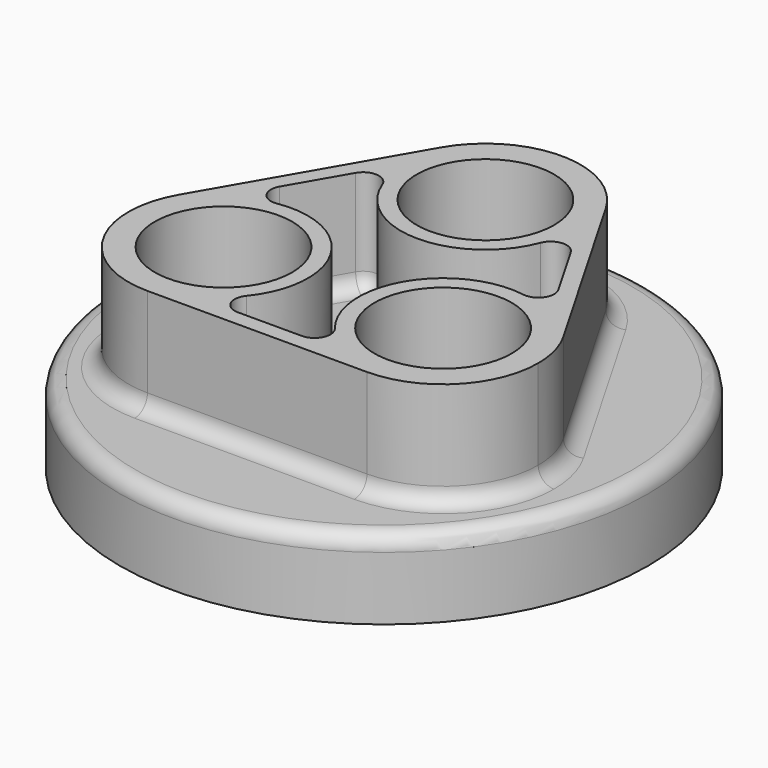
from build123d import *

# Parameters (mm, degrees)
F0_R         = 50
F0_R_2       = 13
F1_DEPTH     = 15
F2_T         = -2.5
F3_DEPTH     = 20
F4_T         = 3
F4_T3_DEPTH  = 47.5692193817
F4_T5_DEPTH  = 47.5692193817
F4_T7_DEPTH  = 47.5692193817
F4_T18_ANGLE = 120.000000001
F4_T20_ANGLE = 120.000000001
F4_T22_ANGLE = 120.000000001
F5_R         = 3


# Not quite as in the source:
# - two fillets or chamfers of one size are made in one step
# - a shell that OpenCascade refuses in one call is made with other operations: the cavity is built on its own and cut out


with BuildPart() as f1:
    # F0 (on Top) → F1 (new body)
    with BuildSketch(Plane.XY):
        Circle(F0_R)
        with BuildLine():
            ThreePointArc((-20.7846096908, -30), (-36.3730669589, -21), (-36.3730669589, -3))
            Line((-36.3730669589, -3), (-15.5884572681, 33))
            ThreePointArc((-15.5884572681, 33), (0, 42), (15.5884572681, 33))
            Line((15.5884572681, 33), (36.3730669589, -3))
            ThreePointArc((36.3730669589, -3), (38.171274564, -7.3412571882), (38.7846096908, -12))
            ThreePointArc((38.7846096908, -12), (33.5125317522, -24.7279220614), (20.7846096908, -30))
            Line((20.7846096908, -30), (-20.7846096908, -30))
        make_face(mode=Mode.SUBTRACT)
        with BuildLine():
            ThreePointArc((-20.7846096908, -30), (-8.0566876295, -24.7279220614), (-2.7846096908, -12))
            ThreePointArc((-2.7846096908, -12), (-16.125866879, 5.3866648732), (-36.3730669589, -3))
            ThreePointArc((-36.3730669589, -3), (-36.3730669589, -21), (-20.7846096908, -30))
        make_face()
        with Locations((-20.7846096908, -12)):
            Circle(F0_R_2, mode=Mode.SUBTRACT)
        with BuildLine():
            ThreePointArc((15.5884572681, 33), (0, 42), (-15.5884572681, 33))
            ThreePointArc((-15.5884572681, 33), (-4.6587428118, 6.6133351268), (18, 24))
            ThreePointArc((18, 24), (17.3866648732, 28.6587428118), (15.5884572681, 33))
        make_face()
        with Locations((0, 24)):
            Circle(F0_R_2, mode=Mode.SUBTRACT)
        with BuildLine():
            ThreePointArc((36.3730669589, -3), (5.1961524227, -3), (20.7846096908, -30))
            ThreePointArc((20.7846096908, -30), (33.5125317522, -24.7279220614), (38.7846096908, -12))
            ThreePointArc((38.7846096908, -12), (38.171274564, -7.3412571882), (36.3730669589, -3))
        make_face()
        with Locations((20.7846096908, -12)):
            Circle(F0_R_2, mode=Mode.SUBTRACT)
        with BuildLine():
            ThreePointArc((-36.3730669589, -3), (-16.125866879, 5.3866648732), (-2.7846096908, -12))
            ThreePointArc((-2.7846096908, -12), (-8.0566876295, -24.7279220614), (-20.7846096908, -30))
            Line((-20.7846096908, -30), (20.7846096908, -30))
            ThreePointArc((20.7846096908, -30), (5.1961524227, -3), (36.3730669589, -3))
            Line((36.3730669589, -3), (15.5884572681, 33))
            ThreePointArc((15.5884572681, 33), (17.3866648732, 28.6587428118), (18, 24))
            ThreePointArc((18, 24), (-4.6587428118, 6.6133351268), (-15.5884572681, 33))
            Line((-15.5884572681, 33), (-36.3730669589, -3))
        make_face()
    extrude(amount=-F1_DEPTH)

    # F2
    f2_openings = [f1.faces().sort_by_distance(p)[0] for p in [
        (0, 0, -15),
    ]]
    offset(amount=F2_T, openings=f2_openings)

    # F0 (on Top) → F3 (join)
    with BuildSketch(Plane.XY):
        with BuildLine():
            ThreePointArc((15.5884572681, 33), (0, 42), (-15.5884572681, 33))
            ThreePointArc((-15.5884572681, 33), (-4.6587428118, 6.6133351268), (18, 24))
            ThreePointArc((18, 24), (17.3866648732, 28.6587428118), (15.5884572681, 33))
        make_face()
        with Locations((0, 24)):
            Circle(F0_R_2, mode=Mode.SUBTRACT)
        with BuildLine():
            ThreePointArc((-20.7846096908, -30), (-8.0566876295, -24.7279220614), (-2.7846096908, -12))
            ThreePointArc((-2.7846096908, -12), (-16.125866879, 5.3866648732), (-36.3730669589, -3))
            ThreePointArc((-36.3730669589, -3), (-36.3730669589, -21), (-20.7846096908, -30))
        make_face()
        with Locations((-20.7846096908, -12)):
            Circle(F0_R_2, mode=Mode.SUBTRACT)
        with BuildLine():
            ThreePointArc((36.3730669589, -3), (5.1961524227, -3), (20.7846096908, -30))
            ThreePointArc((20.7846096908, -30), (33.5125317522, -24.7279220614), (38.7846096908, -12))
            ThreePointArc((38.7846096908, -12), (38.171274564, -7.3412571882), (36.3730669589, -3))
        make_face()
        with Locations((20.7846096908, -12)):
            Circle(F0_R_2, mode=Mode.SUBTRACT)
        with BuildLine():
            ThreePointArc((-36.3730669589, -3), (-16.125866879, 5.3866648732), (-2.7846096908, -12))
            ThreePointArc((-2.7846096908, -12), (-8.0566876295, -24.7279220614), (-20.7846096908, -30))
            Line((-20.7846096908, -30), (20.7846096908, -30))
            ThreePointArc((20.7846096908, -30), (5.1961524227, -3), (36.3730669589, -3))
            Line((36.3730669589, -3), (15.5884572681, 33))
            ThreePointArc((15.5884572681, 33), (17.3866648732, 28.6587428118), (18, 24))
            ThreePointArc((18, 24), (-4.6587428118, 6.6133351268), (-15.5884572681, 33))
            Line((-15.5884572681, 33), (-36.3730669589, -3))
        make_face()
    extrude(amount=F3_DEPTH)

    # F4: shell of thickness 3, made by hand


with BuildPart() as f4_core1:
    # F4_t2: copy of F1
    add(f1.part)

    # the walls: a layer under each face that stays
    f4_faces = [f4_core1.faces().sort_by_distance(p)[0] for p in [
        (-50, 0, -7.5),
        (-46.6666666667, -13.3333333333, -15),
        (-47.5, 0, -8.75),
        (0, 0, -2.5),
        (-15.5, 24, -8.75),
        (-10.3333333333, 13.6666666667, -15),
        (-13, 24, 2.5),
        (7.7846096908, -12, 2.5),
        (10.4512763575, -22.3333333333, -15),
        (-33.7846096908, -12, 2.5),
        (-31.1179430242, -22.3333333333, -15),
        (25.9807621135, 15, 10),
        (36.3730669589, -21, 10),
        (0, -30, 10),
        (-36.3730669589, -21, 10),
        (-25.9807621135, 15, 10),
        (0, 42, 10),
        (-36.2846096908, -12, -8.75),
        (5.2846096908, -12, -8.75),
        (-33.3333333333, -33.3333333333, 0),
    ]]
    thicken(f4_faces, amount=-F4_T, mode=Mode.SUBTRACT)

    # F4_s4 → F4_t3 (cut)
    with BuildSketch(Plane(origin=(11.8923048454, -20.5980762114, 0), x_dir=(0, 0, 1), z_dir=(-0.5, 0.8660254038, 0))):
        Polygon((0.03, 30.03), (0, 27), (-3, 27), (-3, 30), align=None)
    extrude(amount=F4_T3_DEPTH, mode=Mode.SUBTRACT)

    # F4_s6 → F4_t5 (cut)
    with BuildSketch(Plane.YZ.offset(-23.7846096908)):
        Polygon((-30.03, 0.03), (-27, 0), (-27, -3), (-30, -3), align=None)
    extrude(amount=F4_T5_DEPTH, mode=Mode.SUBTRACT)

    # F4_s8 → F4_t7 (cut)
    with BuildSketch(Plane(origin=(11.8923048454, 20.5980762114, 0), x_dir=(0, 0, 1), z_dir=(-0.5, -0.8660254038, 0))):
        Polygon((0.03, 30.03), (0, 27), (-3, 27), (-3, 30), align=None)
    extrude(amount=F4_T7_DEPTH, mode=Mode.SUBTRACT)

    # F4_s9 → F4_t10 (revolve, cut)
    with BuildSketch(Plane.XZ):
        Polygon((47.47, -2.53), (50.5, -2.5), (50.5, 0.5), (47.5, 0.5), align=None)
    revolve(axis=Axis((0, 0, -2.5), (0, 0, 1)), mode=Mode.SUBTRACT)

    # F4_s11 → F4_t12 (revolve, cut)
    with BuildSketch(Plane.XZ.offset(12)):
        Polygon((36.3146096908, -2.53), (36.2846096908, 0.5), (33.2846096908, 0.5), (33.2846096908, -2.5), align=None)
    revolve(axis=Axis((20.7846096908, -12, -2.5), (0, 0, 1)), mode=Mode.SUBTRACT)

    # F4_s13 → F4_t14 (revolve, cut)
    with BuildSketch(Plane.XZ.offset(12)):
        Polygon((-5.2546096908, -2.53), (-5.2846096908, 0.5), (-8.2846096908, 0.5), (-8.2846096908, -2.5), align=None)
    revolve(axis=Axis((-20.7846096908, -12, -2.5), (0, 0, 1)), mode=Mode.SUBTRACT)

    # F4_s15 → F4_t16 (revolve, cut)
    with BuildSketch(Plane.XZ.offset(-24)):
        Polygon((15.53, -2.53), (15.5, 0.5), (12.5, 0.5), (12.5, -2.5), align=None)
    revolve(axis=Axis((0, 24, -2.5), (0, 0, 1)), mode=Mode.SUBTRACT)

    # F4_s17 → F4_t18 (revolve, cut)
    with BuildSketch(Plane.YZ.offset(20.7846096908)):
        Polygon((-30.03, 0.03), (-27, 0), (-27, -3), (-30, -3), align=None)
    revolve(axis=Axis((20.7846096908, -12, 0), (0, 0, 1)), revolution_arc=F4_T18_ANGLE, mode=Mode.SUBTRACT)

    # F4_s19 → F4_t20 (revolve, cut)
    with BuildSketch(Plane(origin=(-10.3923048454, -18, 0), x_dir=(0, 0, 1), z_dir=(0.5, 0.8660254038, 0))):
        Polygon((0.03, -30.03), (0, -27), (-3, -27), (-3, -30), align=None)
    revolve(axis=Axis((-20.7846096908, -12, 0), (0, 0, 1)), revolution_arc=F4_T20_ANGLE, mode=Mode.SUBTRACT)

    # F4_s21 → F4_t22 (revolve, cut)
    with BuildSketch(Plane(origin=(-10.3923048454, 18, 0), x_dir=(0, 0, 1), z_dir=(0.5, -0.8660254038, 0))):
        Polygon((0.03, -30.03), (0, -27), (-3, -27), (-3, -30), align=None)
    revolve(axis=Axis((0, 24, 0), (0, 0, 1)), revolution_arc=F4_T22_ANGLE, mode=Mode.SUBTRACT)


with BuildPart() as f1_1:
    add(f1.part)

    # what is left inside the walls is the cavity
    f4_cavity = [f4_core1.part.solids().sort_by_distance(p)[0] for p in [
        (6.902222, -3.985, 13.5),
    ]]
    add(f4_cavity, mode=Mode.SUBTRACT)

    # F5
    f5_edges = [f1_1.edges().sort_by_distance(p)[0] for p in [
        (-47.5, 0, -2.5),
        (5.28461, -12, -2.5),
        (-36.28461, -12, -2.5),
        (-15.5, 24, -2.5),
        (6.928203, -4, 0.5),
        (23.382686, 13.5, 0.5),
        (0, 8, 0.5),
        (-23.382686, 13.5, 0.5),
        (-6.928203, -4, 0.5),
        (0, -27, 0.5),
        (0, -30, 0),
        (-50, 0, 0),
        (0, 42, 0),
        (-25.980762, 15, 0),
        (-36.373067, -21, 0),
        (36.373067, -21, 0),
        (25.980762, 15, 0),
        (-15.216845, -27, 10.25),
        (15.216845, -27, 10.25),
        (30.991109, 0.321825, 10.25),
        (15.774263, 26.678175, 10.25),
        (-15.774263, 26.678175, 10.25),
        (-30.991109, 0.321825, 10.25),
    ]]
    fillet(f5_edges, radius=F5_R)


solid = f1_1.part
